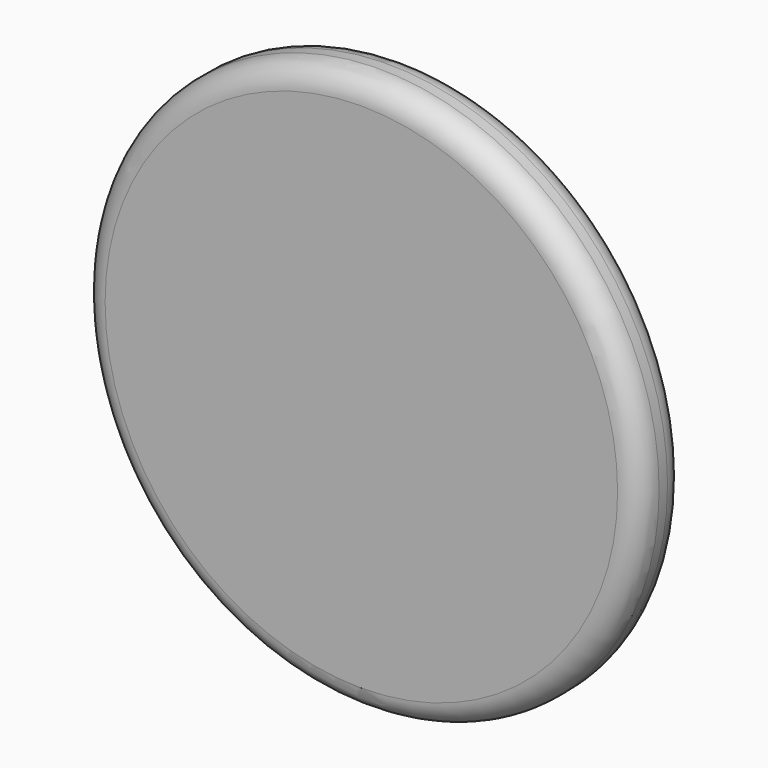
from build123d import *

# Parameters (mm, degrees)
F0_R     = 37.9906163482
F1_DEPTH = 7.7
F2_R     = 3.138


# Not quite as in the source:
# - the program builds the solid bodies; features that only make, move or delete a surface that nothing else refers to are left out


with BuildPart() as f1:
    # F0 (on Front) → F1 (new body)
    with BuildSketch(Plane.XZ):
        Circle(F0_R)
    extrude(amount=F1_DEPTH)

    # F2
    f2_edges = [f1.edges().sort_by_distance(p)[0] for p in [
        (37.990616, -3.85, 0),
        (-37.990616, 0, 0),
        (-37.990616, -7.7, 0),
    ]]
    fillet(f2_edges, radius=F2_R)


solid = f1.part
